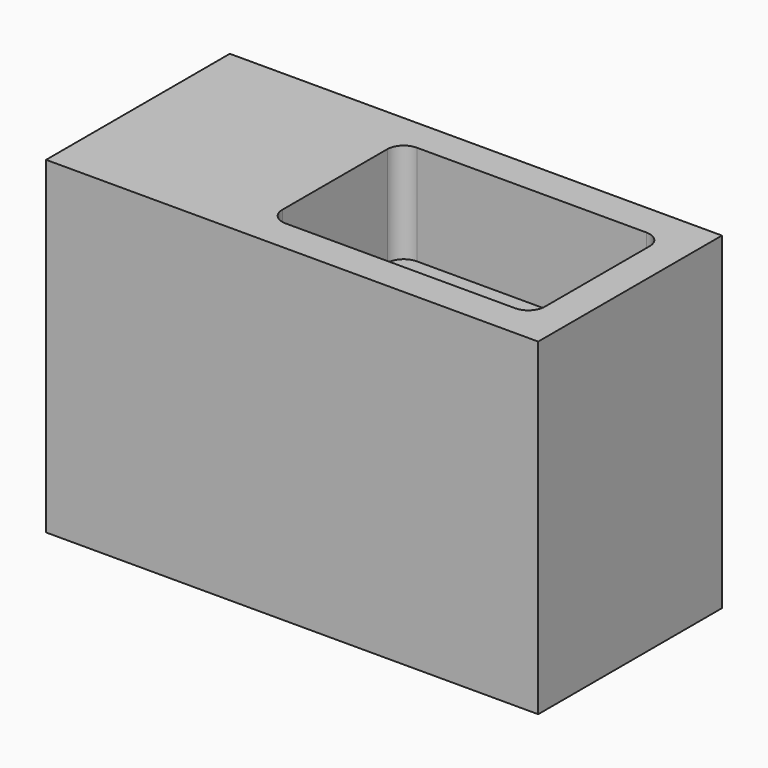
from build123d import *

# Parameters (mm, degrees)
F0_W         = 1500
F0_H         = 700
F1_DEPTH     = 1000
F3_DEPTH     = 305
F4_TEXT_SIZE = 85.6802381979
F5_DEPTH     = 33


# Not quite as in the source:
# - Text() gives the source's letters only with a copy of the font that has no kerning and outlines rounded to 1/6400 em; it was checked with that copy


with BuildPart() as f1:
    # F0 (on Top) → F1 (new body)
    with BuildSketch(Plane.XY):
        Rectangle(F0_W, F0_H)
    extrude(amount=F1_DEPTH)

    # F2 (on face) → F3 (cut)
    with BuildSketch(Plane.XY.offset(1000)):
        with BuildLine():
            Line((-100, -250), (600, -250))
            ThreePointArc((600, -250), (635.3553390593, -235.3553390593), (650, -200))
            Line((650, -200), (650, 200))
            ThreePointArc((650, 200), (635.3553390593, 235.3553390593), (600, 250))
            Line((600, 250), (-100, 250))
            ThreePointArc((-100, 250), (-135.3553390593, 235.3553390593), (-150, 200))
            Line((-150, 200), (-150, -200))
            ThreePointArc((-150, -200), (-135.3553390593, -235.3553390593), (-100, -250))
        make_face()
    extrude(amount=-F3_DEPTH, mode=Mode.SUBTRACT)

    # F4 (on face) → F5 (cut)
    with BuildSketch(Plane.XY.offset(695)):
        with Locations((-100, 138.3102284975)):
            Text('TRIMMER & SINK', F4_TEXT_SIZE, font='Open Sans', text_align=(TextAlign.LEFT, TextAlign.BOTTOM))
    extrude(amount=-F5_DEPTH, mode=Mode.SUBTRACT)


solid = f1.part
